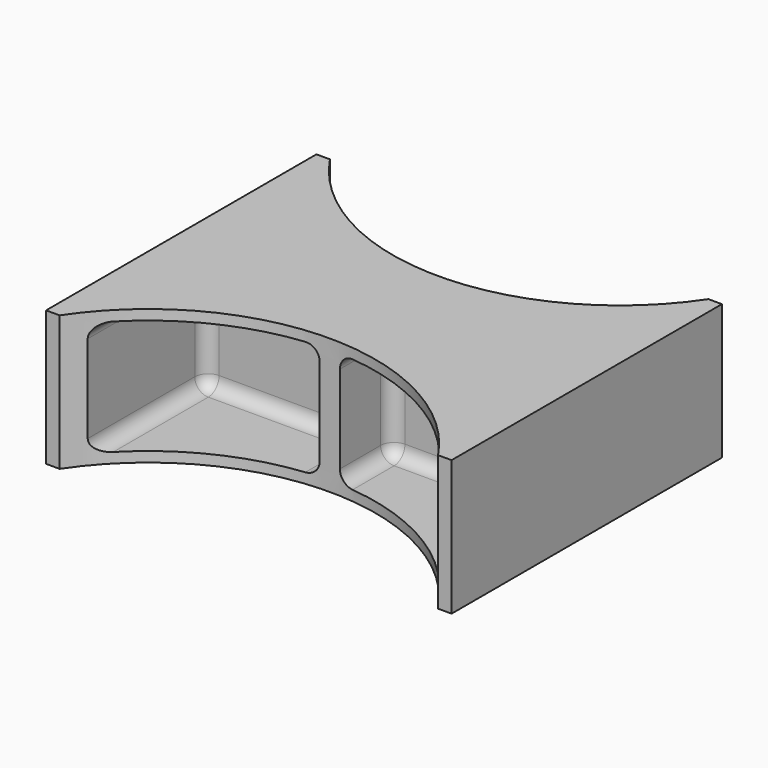
from build123d import *

# Parameters (mm, degrees)
F0_W     = 152.4
F0_H     = 127
F1_DEPTH = 50.8
F3_DEPTH = 50.801
F5_W     = 62.23
F5_H     = 43.18
F6_DEPTH = 62.231
F7_F1_R  = 5.08
F7_F2_R  = 5.08
F7_F3_R  = 5.08
F7_F4_R  = 5.08
F7_F5_R  = 5.08
F7_F6_R  = 5.08
F7_F7_R  = 5.08
F7_F8_R  = 5.08
F7_F9_R  = 5.08
F7_F10_R = 5.08
F7_F11_R = 5.08
F7_F12_R = 5.08
F7_F13_R = 5.08
F7_F14_R = 5.08
F7_F15_R = 5.08
F7_F16_R = 5.08


# Not quite as in the source:
# - a pattern or mirror of a feature is missing from the dataset's text; its kind, count and spacing are read off the source's solid


with BuildPart() as f1:
    # F0 (on Top) → F1 (new body)
    with BuildSketch(Plane.XY):
        Rectangle(F0_W, F0_H)
    extrude(amount=F1_DEPTH)

    # F2 (on face) → F3 (cut, through all)
    with BuildSketch(Plane.XY.offset(50.8)):
        with BuildLine():
            Line((-71.12, -63.5), (71.12, -63.5))
            ThreePointArc((71.12, -63.5), (0, -25.4), (-71.12, -63.5))
        make_face()
        with BuildLine():
            ThreePointArc((-71.12, 63.5), (0, 25.4), (71.12, 63.5))
            Line((71.12, 63.5), (-71.12, 63.5))
        make_face()
    extrude(amount=-F3_DEPTH, mode=Mode.SUBTRACT)

    # F5 (on offset) → F6 (cut, through all)
    with BuildSketch(Plane.XZ.offset(1.27)):
        with Locations((-34.925, 25.4)):
            Rectangle(F5_W, F5_H)
        with Locations((34.925, 25.4)):
            Rectangle(F5_W, F5_H)
    f6 = extrude(amount=F6_DEPTH, mode=Mode.SUBTRACT)

    # F6_copies: F6 across plane
    add(f6.mirror(Plane.ZX), mode=Mode.SUBTRACT)

    # F7: fillet of radius 5.08 on 28 edges, made by hand

    # F7_f1
    f7_f1_edges = [f1.edges().sort_by_distance(p)[0] for p in [
        (34.925, -1.27, 3.81),
    ]]
    fillet(f7_f1_edges, radius=F7_F1_R)

    # F7_f2
    f7_f2_edges = [f1.edges().sort_by_distance(p)[0] for p in [
        (66.04, -31.4933212262, 3.81),
    ]]
    fillet(f7_f2_edges, radius=F7_F2_R)

    # F7_f3
    f7_f3_edges = [f1.edges().sort_by_distance(p)[0] for p in [
        (3.81, -15.9175013231, 3.81),
    ]]
    fillet(f7_f3_edges, radius=F7_F3_R)

    # F7_f4
    f7_f4_edges = [f1.edges().sort_by_distance(p)[0] for p in [
        (3.81, -15.9175013231, 46.99),
    ]]
    fillet(f7_f4_edges, radius=F7_F4_R)

    # F7_f5
    f7_f5_edges = [f1.edges().sort_by_distance(p)[0] for p in [
        (-34.925, -1.27, 3.81),
    ]]
    fillet(f7_f5_edges, radius=F7_F5_R)

    # F7_f6
    f7_f6_edges = [f1.edges().sort_by_distance(p)[0] for p in [
        (-3.81, -15.9175013231, 3.81),
    ]]
    fillet(f7_f6_edges, radius=F7_F6_R)

    # F7_f7
    f7_f7_edges = [f1.edges().sort_by_distance(p)[0] for p in [
        (-66.04, -31.4933212262, 3.81),
    ]]
    fillet(f7_f7_edges, radius=F7_F7_R)

    # F7_f8
    f7_f8_edges = [f1.edges().sort_by_distance(p)[0] for p in [
        (-66.04, -31.4933212262, 46.99),
    ]]
    fillet(f7_f8_edges, radius=F7_F8_R)

    # F7_f9
    f7_f9_edges = [f1.edges().sort_by_distance(p)[0] for p in [
        (-3.81, 1.27, 25.4),
    ]]
    fillet(f7_f9_edges, radius=F7_F9_R)

    # F7_f10
    f7_f10_edges = [f1.edges().sort_by_distance(p)[0] for p in [
        (-37.465, 1.27, 46.99),
    ]]
    fillet(f7_f10_edges, radius=F7_F10_R)

    # F7_f11
    f7_f11_edges = [f1.edges().sort_by_distance(p)[0] for p in [
        (-66.04, 31.4933212262, 46.99),
    ]]
    fillet(f7_f11_edges, radius=F7_F11_R)

    # F7_f12
    f7_f12_edges = [f1.edges().sort_by_distance(p)[0] for p in [
        (-66.04, 31.4933212262, 3.81),
    ]]
    fillet(f7_f12_edges, radius=F7_F12_R)

    # F7_f13
    f7_f13_edges = [f1.edges().sort_by_distance(p)[0] for p in [
        (34.925, 1.27, 3.81),
    ]]
    fillet(f7_f13_edges, radius=F7_F13_R)

    # F7_f14
    f7_f14_edges = [f1.edges().sort_by_distance(p)[0] for p in [
        (66.04, 31.4933212262, 3.81),
    ]]
    fillet(f7_f14_edges, radius=F7_F14_R)

    # F7_f15
    f7_f15_edges = [f1.edges().sort_by_distance(p)[0] for p in [
        (66.04, 31.4933212262, 46.99),
    ]]
    fillet(f7_f15_edges, radius=F7_F15_R)

    # F7_f16
    f7_f16_edges = [f1.edges().sort_by_distance(p)[0] for p in [
        (3.81, 1.27, 25.4),
    ]]
    fillet(f7_f16_edges, radius=F7_F16_R)


solid = f1.part
